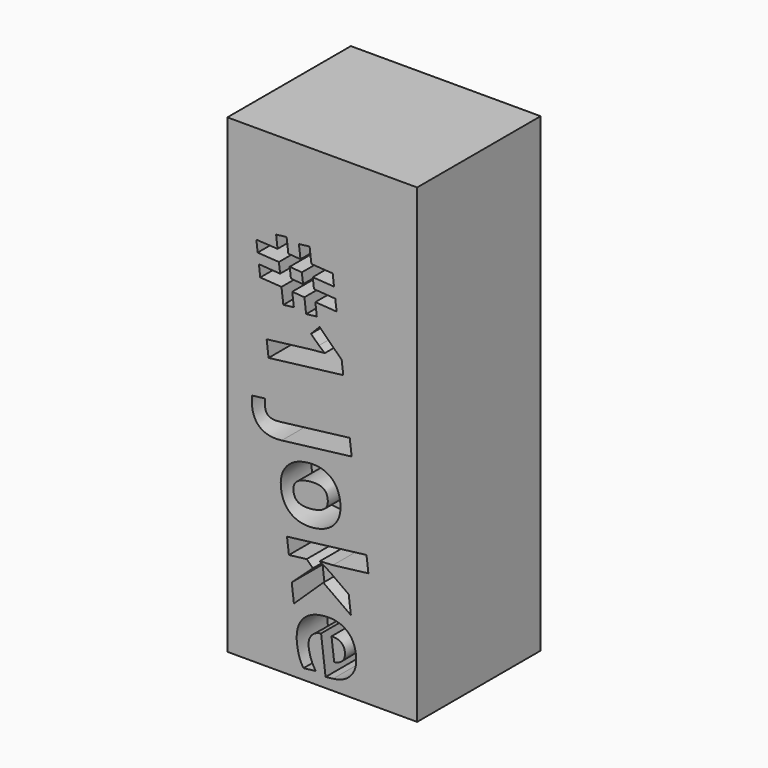
from build123d import *

# Parameters (mm, degrees)
F0_W         = 62.4676980078
F0_H         = 154.8856720328
F1_DEPTH     = 50.8
F2_TEXT_SIZE = 34.7024165315
F3_DEPTH     = 12.7


# Not quite as in the source:
# - Text() gives the source's letters only with a copy of the font that has no kerning and outlines rounded to 1/6400 em; it was checked with that copy


with BuildPart() as f1:
    # F0 (on Front) → F1 (new body)
    with BuildSketch(Plane.XZ):
        with Locations((-7.5588766485, -1.7114467919)):
            Rectangle(F0_W, F0_H)
    extrude(amount=F1_DEPTH)

    # F2 (on face) → F3 (cut)
    with BuildSketch(Plane.XZ.offset(50.8)):
        with Locations(Location((-29.6869133013, 46.9130270383), (0, 0, -83.0518271621))):
            Text('#1 Joke', F2_TEXT_SIZE, font='Open Sans', font_style=FontStyle.BOLD, text_align=(TextAlign.LEFT, TextAlign.BOTTOM))
    extrude(amount=-F3_DEPTH, mode=Mode.SUBTRACT)


solid = f1.part
